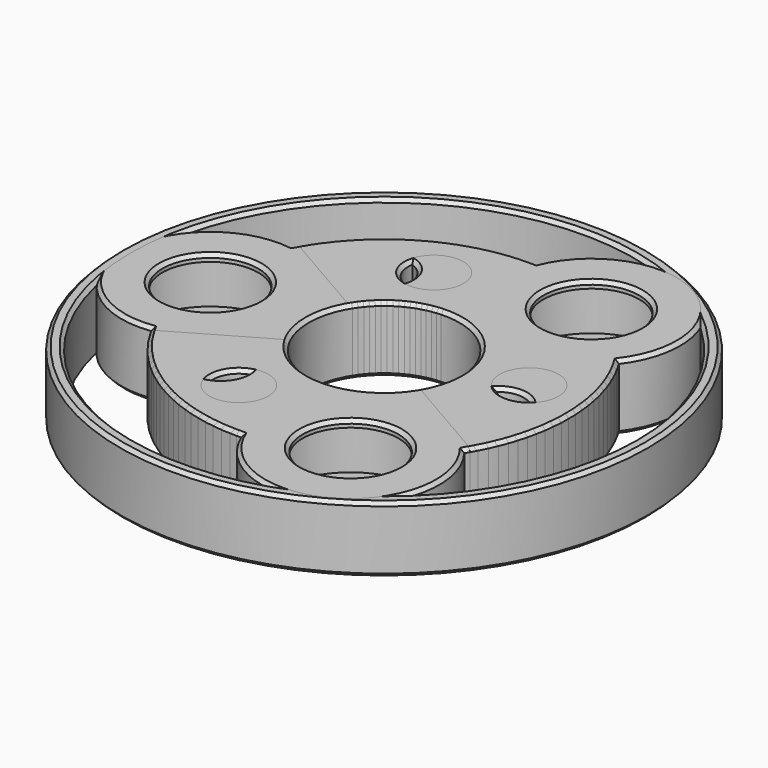
from build123d import *

# Parameters (mm, degrees)
F0_R     = 3.81
F0_R_2   = 7
F1_DEPTH = 4.826
F2_R     = 10.605
F3_DEPTH = 3.81
F4_SIZE  = 0.508
F5_R     = 38.5777676135
F5_R_2   = 36.5333929687
F6_DEPTH = 4.826
F7_COUNT = 3
F8_SIZE  = 0.508


# Not quite as in the source:
# - a feature names something its author has since deleted; it is built from what else it names


with BuildPart() as f1:
    # F0 (on Top) → F1 (new body, symmetric)
    with BuildSketch(Plane.XY):
        with BuildLine():
            ThreePointArc((0, -11), (-11, 0), (0, 11))
            Line((0, 11), (0, 15.1155683379))
            Line((0, 15.1155683379), (0, 24.3954310155))
            Line((0, 24.3954310155), (0, 27.0066420172))
            ThreePointArc((0, 27.0066420172), (-13.8145365452, 23.2059753746), (-23.7408112179, 12.8737172473))
            ThreePointArc((-23.7408112179, 12.8737172473), (-38.380196577, 0), (-23.7408112179, -12.8737172473))
            ThreePointArc((-23.7408112179, -12.8737172473), (-13.8145365452, -23.2059753746), (0, -27.0066420172))
            Line((0, -27.0066420172), (0, -24.3954310155))
            Line((0, -24.3954310155), (0, -15.1155683379))
            Line((0, -15.1155683379), (0, -11))
        make_face()
        with Locations((-11.9443507897, -14.9462528673)):
            Circle(F0_R, mode=Mode.SUBTRACT)
        with Locations((-25.4, 0)):
            Circle(F0_R_2, mode=Mode.SUBTRACT)
        with Locations((-11.9443507897, 14.9462528673)):
            Circle(F0_R, mode=Mode.SUBTRACT)
    extrude(amount=F1_DEPTH, both=True)

    # F2 (on Top) → F3 (cut, symmetric)
    with BuildSketch(Plane.XY):
        with Locations((-25.4, 0)):
            Circle(F2_R)
    extrude(amount=F3_DEPTH, both=True, mode=Mode.SUBTRACT)

    # F4
    f4_edges = [f1.edges().sort_by_distance(p)[0] for p in [
        (-11, 0, -4.826),
        (-11, 0, 4.826),
        (-32.4, 0, -4.826),
        (-32.4, 0, 4.826),
        (-13.814537, 23.205975, -4.826),
        (-13.814537, 23.205975, 4.826),
        (-38.380197, 0, 4.826),
        (-13.814537, -23.205975, 4.826),
        (-38.380197, 0, -4.826),
        (-13.814537, -23.205975, -4.826),
        (-15.754351, -14.946253, -4.826),
        (-15.754351, 14.946253, -4.826),
        (-15.754351, -14.946253, 4.826),
        (-15.754351, 14.946253, 4.826),
    ]]
    chamfer(f4_edges, length=F4_SIZE)


with BuildPart() as f6:
    # F5 (on Top) → F6 (new body, symmetric)
    with BuildSketch(Plane.XY):
        Circle(F5_R)
        Circle(F5_R_2, mode=Mode.SUBTRACT)
    extrude(amount=F6_DEPTH, both=True)

    # F8
    f8_edges = [f6.edges().sort_by_distance(p)[0] for p in [
        (-38.577768, 0, 4.826),
        (-36.533393, 0, 4.826),
        (-38.577768, 0, -4.826),
        (-36.533393, 0, -4.826),
    ]]
    chamfer(f8_edges, length=F8_SIZE)


with BuildPart() as f7_1:
    # F7: instance of F1
    add(f1.part.rotate(Axis((0, 0, 0), (0, 0, 1)), 1 * 360 / F7_COUNT))


with BuildPart() as f7_2:
    # F7: instance of F1
    add(f1.part.rotate(Axis((0, 0, 0), (0, 0, 1)), 2 * 360 / F7_COUNT))


solid = Compound([f1.part, f6.part, f7_1.part, f7_2.part])
